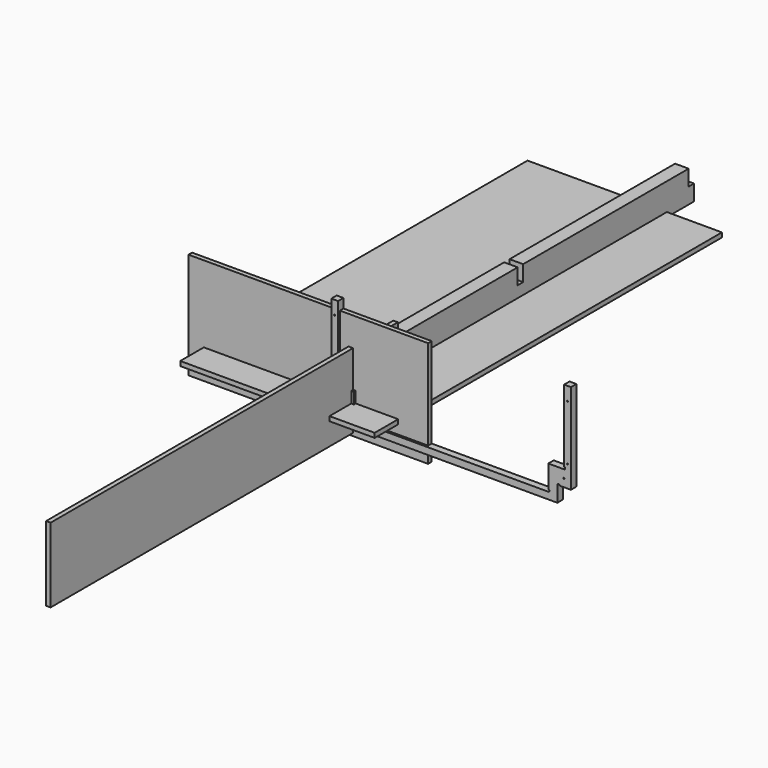
from build123d import *

# Parameters (mm, degrees)
F0_R      = 1.5875
F1_DEPTH  = 19.05
F2_W      = 38.1
F2_H      = 88.9
F3_DEPTH  = 1219.2
F4_W      = 19.05
F4_H      = 44.45
F5_DEPTH  = 50.8
F7_W      = 19.05
F7_H      = 44.45
F8_DEPTH  = 50.8
F9_W      = 673.1
F9_H      = 298.45
F10_DEPTH = 12.7
F11_W     = 1219.2
F11_H     = 209.55
F12_DEPTH = 12.7
F13_W     = 546.1
F13_H     = 1219.2
F14_DEPTH = 12.7


# Not quite as in the source:
# - a pattern or mirror of a feature is missing from the dataset's text; its kind, count and spacing are read off the source's solid


with BuildPart() as f1:
    # F0 (on Front) → F1 (new body)
    with BuildSketch(Plane.XZ):
        with BuildLine():
            Line((-5.3433722377, 44.45), (-24.3933722377, 44.45))
            ThreePointArc((-24.3933722377, 44.45), (-27.5683722377, 47.625), (-24.3933722377, 50.8))
            Line((-24.3933722377, 50.8), (-24.3933722377, 254))
            Line((-24.3933722377, 254), (-43.4433722377, 254))
            Line((-43.4433722377, 254), (-43.4433722377, 44.45))
            Line((-43.4433722377, 44.45), (-43.4433722377, 0))
            Line((-43.4433722377, 0), (-11.6933722377, 0))
            ThreePointArc((-11.6933722377, 0), (-8.5183722377, 3.175), (-5.3433722377, 0))
            Line((-5.3433722377, 0), (-5.3433722377, -44.45))
            Line((-5.3433722377, -44.45), (293.1066277623, -44.45))
            Line((293.1066277623, -44.45), (591.5566277623, -44.45))
            Line((591.5566277623, -44.45), (591.5566277623, 0))
            ThreePointArc((591.5566277623, 0), (594.7316277623, 3.175), (597.9066277623, 0))
            Line((597.9066277623, 0), (629.6566277623, 0))
            Line((629.6566277623, 0), (629.6566277623, 44.45))
            Line((629.6566277623, 44.45), (629.6566277623, 254))
            Line((629.6566277623, 254), (610.6066277623, 254))
            Line((610.6066277623, 254), (610.6066277623, 50.8))
            ThreePointArc((610.6066277623, 50.8), (613.7816277623, 47.625), (610.6066277623, 44.45))
            Line((610.6066277623, 44.45), (591.5566277623, 44.45))
            Line((591.5566277623, 44.45), (566.1566277623, 44.45))
            Line((566.1566277623, 44.45), (566.1566277623, -19.05))
            ThreePointArc((566.1566277623, -19.05), (569.3316277623, -22.225), (566.1566277623, -25.4))
            Line((566.1566277623, -25.4), (293.1066277623, -25.4))
            Line((293.1066277623, -25.4), (20.0566277623, -25.4))
            ThreePointArc((20.0566277623, -25.4), (16.8816277623, -22.225), (20.0566277623, -19.05))
            Line((20.0566277623, -19.05), (20.0566277623, 44.45))
            Line((20.0566277623, 44.45), (-5.3433722377, 44.45))
        make_face()
        with Locations((-23.7429365516, 22.225)):
            Circle(F0_R, mode=Mode.SUBTRACT)
        with Locations((-33.9183722377, 60.6392584741)):
            Circle(F0_R, mode=Mode.SUBTRACT)
        with Locations((609.9561920762, 22.225)):
            Circle(F0_R, mode=Mode.SUBTRACT)
        with Locations((620.1316277623, 60.6392584741)):
            Circle(F0_R, mode=Mode.SUBTRACT)
        with Locations((-33.9183722377, 215.9)):
            Circle(F0_R, mode=Mode.SUBTRACT)
        with Locations((620.1316277623, 215.9)):
            Circle(F0_R, mode=Mode.SUBTRACT)
    extrude(amount=F1_DEPTH)


with BuildPart() as f3:
    # F2 (on Front) → F3 (new body)
    with BuildSketch(Plane.XZ):
        with Locations((-34.1012573361, 44.45)):
            Rectangle(F2_W, F2_H)
    extrude(amount=-F3_DEPTH)

    # F4 (on face) → F5 (cut)
    with BuildSketch(Plane.YZ.offset(-15.0512573361)):
        with Locations((9.525, 66.675)):
            Rectangle(F4_W, F4_H)
    f5 = extrude(amount=-F5_DEPTH, mode=Mode.SUBTRACT)

    # F5_copies: F5 across plane
    add(f5.mirror(Plane.ZX.offset(609.6)), mode=Mode.SUBTRACT)

    # F7 (on face) → F8 (cut)
    with BuildSketch(Plane.YZ.offset(-15.0512573361)):
        with Locations((609.6, 66.675)):
            Rectangle(F7_W, F7_H)
    extrude(amount=-F8_DEPTH, mode=Mode.SUBTRACT)


with BuildPart() as f10:
    # F9 (on Front) → F10 (new body)
    with BuildSketch(Plane.XZ):
        with Locations((-113.032694068, 78.6825154781)):
            Rectangle(F9_W, F9_H)
    extrude(amount=F10_DEPTH)


with BuildPart() as f12:
    # F11 (on Right) → F12 (new body)
    with BuildSketch(Plane.YZ):
        with Locations((-465.0740548134, 42.3955094159)):
            Rectangle(F11_W, F11_H)
    extrude(amount=F12_DEPTH)


with BuildPart() as f14:
    # F13 (on Top) → F14 (new body)
    with BuildSketch(Plane.XY):
        with Locations((-133.4478157043, 514.1422971249)):
            Rectangle(F13_W, F13_H)
    extrude(amount=F14_DEPTH)


solid = Compound([f1.part, f3.part, f10.part, f12.part, f14.part])
